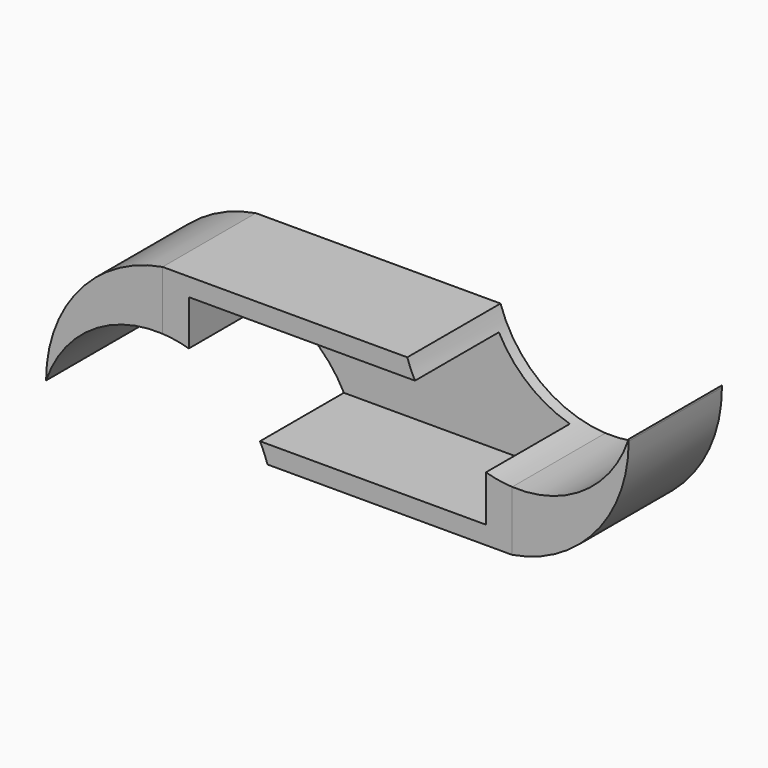
from build123d import *

# Parameters (mm, degrees)
F0_W          = 25.5
F0_H          = 8.9
F1_DEPTH      = 8.9
F2_W          = 30
F2_H          = 12
F2_W_2        = 25.5
F2_H_2        = 8.9
F3_DEPTH      = 10
F4_DEPTH      = 9
F5_DEPTH      = 10
F6_DEPTH      = 10
F9_T1_DEPTH   = 69.160797831
F9_2_T1_DEPTH = 69.160797831
F11_DEPTH     = 10


# Not quite as in the source:
# - a fillet or chamfer that OpenCascade refuses, or shapes differently, is made with other operations: its cross-section is extruded or revolved along the edge and cut away or added


with BuildPart() as f1:
    # F0 (on Top) → F1 (new body)
    with BuildSketch(Plane.XY):
        with Locations((12.75, 4.45)):
            Rectangle(F0_W, F0_H)
    extrude(amount=F1_DEPTH)


with BuildPart() as f3:
    # F2 (on face) → F3 (new body)
    with BuildSketch(Plane.XZ):
        with Locations((12.75, 4.45)):
            Rectangle(F2_W, F2_H)
        with Locations((12.75, 4.45)):
            Rectangle(F2_W_2, F2_H_2, mode=Mode.SUBTRACT)
        with Locations((12.75, 4.45)):
            Rectangle(F2_W_2, F2_H_2)
    extrude(amount=-F3_DEPTH)


with BuildPart() as f4_tool:
    # F4 (cut): a face of the model
    f4_faces = [f1.part.faces().sort_by_distance(p)[0] for p in [
        (12.75, 0, 4.45),
    ]]
    extrude(f4_faces, amount=-F4_DEPTH)


with BuildPart() as f1_1:
    add(f1.part)

    # F4: cut by f4_tool
    add(f4_tool.part, mode=Mode.SUBTRACT)


with BuildPart() as f3_1:
    add(f3.part)

    # F4: cut by f4_tool
    add(f4_tool.part, mode=Mode.SUBTRACT)


with BuildPart() as f5:
    # F5 (new): a face of the model
    f5_faces = [f3_1.part.faces().sort_by_distance(p)[0] for p in [
        (-2.25, 5, 4.45),
    ]]
    extrude(f5_faces, amount=F5_DEPTH)

    # F9: fillet of radius 12 on 1 edges, made by hand

    # F9_s2 → F9_t1 (cut)
    with BuildSketch(Plane.XZ.offset(-39.5803989155)):
        with BuildLine():
            ThreePointArc((-2.25, 10.45), (-9.4151513899, 6.3638071262), (-12.25, -1.3821595662))
            Line((-12.25, -1.3821595662), (-12.25, 10.45))
            Line((-12.25, 10.45), (-2.25, 10.45))
        make_face()
    extrude(amount=F9_T1_DEPTH, mode=Mode.SUBTRACT)


with BuildPart() as f6:
    # F6 (new): a face of the model
    f6_faces = [f3_1.part.faces().sort_by_distance(p)[0] for p in [
        (27.75, 5, 4.45),
    ]]
    extrude(f6_faces, amount=F6_DEPTH)

    # F9#2: fillet of radius 12 on 1 edges, made by hand

    # F9_2_s2 → F9_2_t1 (cut)
    with BuildSketch(Plane.XZ.offset(-39.5803989155)):
        with BuildLine():
            ThreePointArc((27.75, -1.55), (34.9151513899, 2.5361928738), (37.75, 10.2821595662))
            Line((37.75, 10.2821595662), (37.75, -1.55))
            Line((37.75, -1.55), (27.75, -1.55))
        make_face()
    extrude(amount=F9_2_T1_DEPTH, mode=Mode.SUBTRACT)


with BuildPart() as f11_tool:
    # F10 (on face) → F11 (new body)
    with BuildSketch(Plane(origin=(0, 10, 0), x_dir=(-1, 0, 0), z_dir=(0, 1, 0))):
        with BuildLine():
            Line((-27.75, 3.5850068215), (-27.75, 10.45))
            Line((-27.75, 10.45), (-37.75, 10.45))
            ThreePointArc((-37.75, 10.45), (-33.9096848707, 5.3282302527), (-27.75, 3.5850068215))
        make_face()
        with BuildLine():
            ThreePointArc((-27.75, 3.5850068215), (-22.1851807253, 5.6215262811), (-18.75, 10.45))
            Line((-18.75, 10.45), (-27.75, 10.45))
            Line((-27.75, 10.45), (-27.75, 3.5850068215))
        make_face()
        with BuildLine():
            ThreePointArc((-6.75, 29.45), (-13.6275010008, 19.95), (-6.75, 10.45))
            Line((-6.75, 10.45), (-6.75, 29.45))
        make_face()
        with BuildLine():
            Line((2.25, 5.3987446019), (2.25, -1.55))
            Line((2.25, -1.55), (12.25, -1.55))
            Line((12.25, -1.55), (12.25, -1.3821595662))
            ThreePointArc((12.25, -1.3821595662), (8.389860126, 3.6892779702), (2.25, 5.3987446019))
        make_face()
        with BuildLine():
            ThreePointArc((2.25, 5.3987446019), (-3.3337079529, 3.3279886569), (-6.75, -1.55))
            Line((-6.75, -1.55), (2.25, -1.55))
            Line((2.25, -1.55), (2.25, 5.3987446019))
        make_face()
        with BuildLine():
            ThreePointArc((-18.75, -20.55), (-11.8724989992, -11.05), (-18.75, -1.55))
            Line((-18.75, -1.55), (-18.75, -20.55))
        make_face()
    extrude(amount=-F11_DEPTH)


with BuildPart() as f3_2:
    add(f3_1.part)

    # F11: cut by f11_tool
    add(f11_tool.part, mode=Mode.SUBTRACT)


with BuildPart() as f5_1:
    add(f5.part)

    # F11: cut by f11_tool
    add(f11_tool.part, mode=Mode.SUBTRACT)


with BuildPart() as f6_1:
    add(f6.part)

    # F11: cut by f11_tool
    add(f11_tool.part, mode=Mode.SUBTRACT)


solid = Compound([f3_2.part, f5_1.part, f6_1.part])
